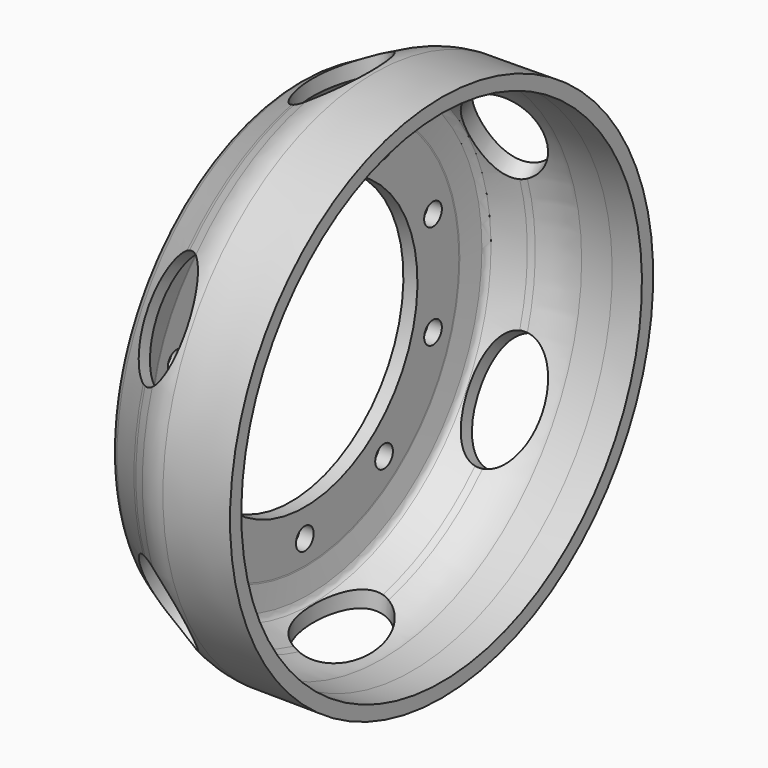
from build123d import *

# Parameters (mm, degrees)
F3_D     = 22
F6_DEPTH = 50
F7_COUNT = 6


# Not quite as in the source:
# - a feature names something its author has since deleted; it is built from what else it names


with BuildPart() as f1:
    # F0 (on Front) → F1 (revolve)
    with BuildSketch(Plane.XZ):
        with BuildLine():
            Line((-14, 140), (0, 140))
            Line((0, 140), (0, 191.403067163))
            ThreePointArc((0, 191.403067163), (0.0221779844, 191.9983451541), (0.0885889717, 192.5903226287))
            Line((0.0885889717, 192.5903226287), (3.5528631489, 215.6749052843))
            ThreePointArc((3.5528631489, 215.6749052843), (4.8479123783, 219.3035139359), (7.4186827987, 222.1731990576))
            Line((7.4186827987, 222.1731990576), (33.1833706576, 235.0529727139))
            ThreePointArc((33.1833706576, 235.0529727139), (35.9660039243, 236.4896966352), (38.7101985287, 237.9985437105))
            ThreePointArc((38.7101985287, 237.9985437105), (56.9739484491, 245.5472492755), (76.530909741, 248.3885134116))
            Line((76.530909741, 248.3885134116), (106.4405143261, 249))
            Line((106.4405143261, 249), (136, 249))
            Line((136, 249), (136, 263))
            Line((136, 263), (68.8061863184, 262.450158596))
            ThreePointArc((68.8061863184, 262.450158596), (55.9691546036, 260.9531474151), (43.7505061927, 256.7418463414))
            Line((43.7505061927, 256.7418463414), (33.5369179607, 251.9357238313))
            ThreePointArc((33.5369179607, 251.9357238313), (31.9160949836, 251.143044942), (30.3198389907, 250.301989801))
            Line((30.3198389907, 250.301989801), (0.2895821372, 233.8977294681))
            ThreePointArc((0.2895821372, 233.8977294681), (-6.516686935, 227.8013589631), (-9.9010395397, 219.3138864616))
            Line((-9.9010395397, 219.3138864616), (-13.6677913562, 194.2137098576))
            ThreePointArc((-13.6677913562, 194.2137098576), (-13.9168325587, 191.9937943279), (-14, 189.7615018613))
            Line((-14, 189.7615018613), (-14, 140))
        make_face()
    revolve(axis=Axis((14.6640119418, 0, 0), (1, 0, 0)))

    # F3 (through all)
    with Locations(Plane(origin=(-14, 0, 0), x_dir=(0, -1, 0), z_dir=(-1, 0, 0))):
        with Locations((0, 167.5), (98.454029759, 135.5103465578), (159.3019664794, 51.7603465578), (159.3019664794, -51.7603465578), (98.454029759, -135.5103465578), (0, -167.5), (-98.454029759, -135.5103465578), (-159.3019664794, -51.7603465578), (-159.3019664794, 51.7603465578), (-98.454029759, 135.5103465578)):
            Hole(F3_D / 2)

    # F5 (on face) → F6 (cut)
    with BuildSketch(Plane.XY.offset(263)):
        with BuildLine():
            add(Edge.make_bspline(
                [(36.5470796824, -55.8635033667), (85.4276441305, -55.8635033667), (60.9873619064, 27.9317516834), (36.5470796824, 111.7270067334), (12.1067974583, 27.9317516834), (-12.3334847658, -55.8635033667), (36.5470796824, -55.8635033667)],
                knots=[0, 0, 0, 2.0943951024, 2.0943951024, 4.1887902048, 4.1887902048, 6.2831853072, 6.2831853072, 6.2831853072], degree=2, weights=[1, 0.5, 1, 0.5, 1, 0.5, 1]))
        make_face()
    f6 = extrude(amount=-F6_DEPTH, mode=Mode.SUBTRACT)

    # F7: F6 ×6 about axis
    f7_axis = Axis((14.6640119418, 0, 0), (1, 0, 0))
    for i in range(1, F7_COUNT):
        add(f6.rotate(f7_axis, i * 360 / F7_COUNT), mode=Mode.SUBTRACT)


solid = f1.part
